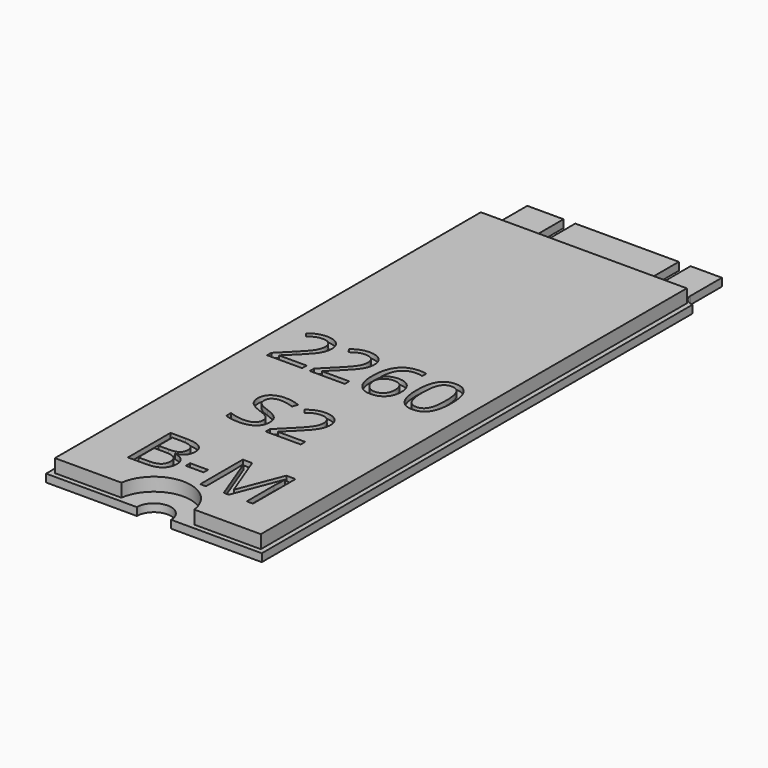
from build123d import *

# Parameters (mm, degrees)
F2_W          = 22
F2_H          = 60
F3_DEPTH      = 0.8
F4_W          = 21
F4_H          = 54.3
F5_DEPTH      = 1.35
F7_DEPTH      = 0.801
F8_R          = 1.75
F9_DEPTH      = 2.151
F11_DEPTH     = 1.35
F12_TEXT_SIZE = 7.6075757129
F13_DEPTH     = 0.5


# Not quite as in the source:
# - Text() gives the source's letters only with a copy of the font that has no kerning and outlines rounded to 1/6400 em; it was checked with that copy


with BuildPart() as f3:
    # F2 (on Top) → F3 (new body)
    with BuildSketch(Plane.XY):
        Rectangle(F2_W, F2_H)
    extrude(amount=F3_DEPTH)

    # F4 (on face) → F5 (join)
    with BuildSketch(Plane.XY.offset(0.8)):
        with Locations((0, -2.35)):
            Rectangle(F4_W, F4_H)
    extrude(amount=F5_DEPTH)

    # F6 (on face) → F7 (cut, through all)
    with BuildSketch(Plane.XY.offset(0.8)):
        with BuildLine():
            Line((-9.925, 26), (-9.925, 30))
            Line((-9.925, 30), (-11, 30))
            Line((-11, 30), (-11, 24.925))
            ThreePointArc((-11, 24.925), (-10.2398602102, 25.2398602102), (-9.925, 26))
        make_face()
        with BuildLine():
            Line((11, 30), (9.925, 30))
            Line((9.925, 30), (9.925, 26))
            ThreePointArc((9.925, 26), (10.2398602102, 25.2398602102), (11, 24.925))
            Line((11, 24.925), (11, 30))
        make_face()
        with BuildLine():
            Line((5.53, 30), (5.53, 26.6))
            ThreePointArc((5.53, 26.6), (6.13, 26), (6.73, 26.6))
            Line((6.73, 26.6), (6.73, 30))
            Line((6.73, 30), (5.53, 30))
        make_face()
        with BuildLine():
            Line((-5.03, 30), (-6.23, 30))
            Line((-6.23, 30), (-6.23, 26.6198236495))
            ThreePointArc((-6.23, 26.6198236495), (-5.63, 26.0198236495), (-5.03, 26.6198236495))
            Line((-5.03, 26.6198236495), (-5.03, 30))
        make_face()
    extrude(amount=-F7_DEPTH, mode=Mode.SUBTRACT)

    # F8 (on face) → F9 (cut, through all)
    with BuildSketch(Plane(origin=(0, 0, 0), x_dir=(1, 0, 0), z_dir=(0, 0, -1))):
        with Locations((0, 30)):
            Circle(F8_R)
    extrude(amount=-F9_DEPTH, mode=Mode.SUBTRACT)

    # F10 (on face) → F11 (cut, through all)
    with BuildSketch(Plane.XY.offset(2.15)):
        with BuildLine():
            ThreePointArc((-1.6770509831, -29.5), (0, -28.25), (1.6770509831, -29.5))
            Line((1.6770509831, -29.5), (3.7165171868, -29.5))
            ThreePointArc((3.7165171868, -29.5), (0, -26.25), (-3.7165171868, -29.5))
            Line((-3.7165171868, -29.5), (-1.6770509831, -29.5))
        make_face()
    extrude(amount=-F11_DEPTH, mode=Mode.SUBTRACT)

    # F12 (on face) → F13 (cut)
    with BuildSketch(Plane.XY.offset(2.15)):
        with Locations((-8.756438514, -5.0887272567)):
            Text('2260', F12_TEXT_SIZE, font='Open Sans', text_align=(TextAlign.LEFT, TextAlign.BOTTOM))
        with Locations((-4.8028765106, -15.4350302262)):
            Text('S2', F12_TEXT_SIZE, font='Open Sans', text_align=(TextAlign.LEFT, TextAlign.BOTTOM))
        with Locations((-6.7796575123, -25.7813331958)):
            Text('B-M', F12_TEXT_SIZE, font='Open Sans', text_align=(TextAlign.LEFT, TextAlign.BOTTOM))
    extrude(amount=-F13_DEPTH, mode=Mode.SUBTRACT)


solid = f3.part
